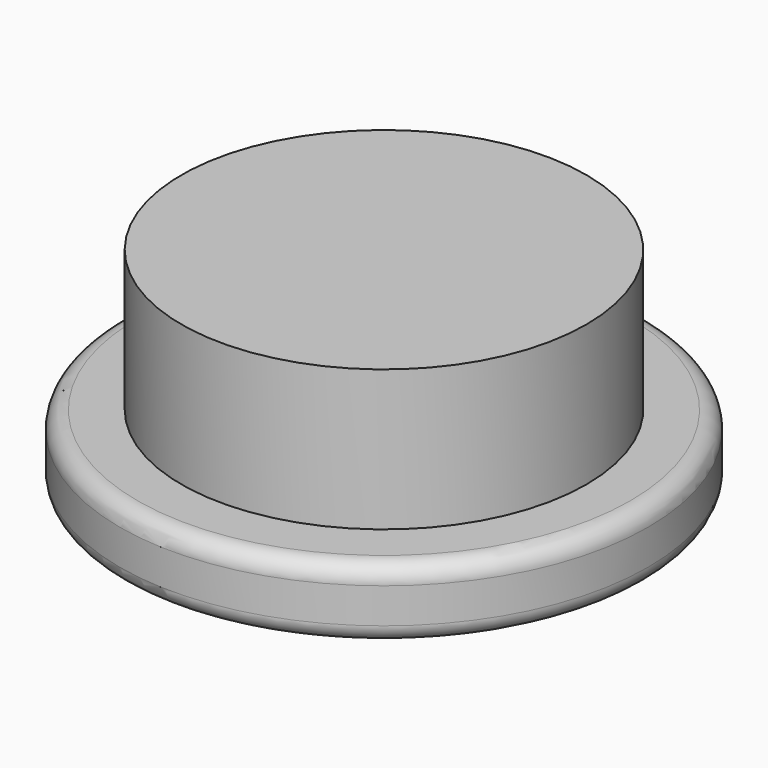
from build123d import *

# Parameters (mm, degrees)
F0_R     = 58.42
F1_DEPTH = 40.64
F2_R     = 76.2
F2_R_2   = 58.42
F3_DEPTH = 20.32
F4_R     = 5.08
F5_DEPTH = 17.78
F7_R     = 25.4
F8_DEPTH = 45.974


with BuildPart() as f1:
    # F0 (on Top) → F1 (new body)
    with BuildSketch(Plane.XY):
        with Locations((-23.1254743153, 3.4657202779)):
            Circle(F0_R)
    extrude(amount=F1_DEPTH)


with BuildPart() as f3:
    # F2 (on face) → F3 (new body)
    with BuildSketch(Plane(origin=(0, 0, 0), x_dir=(1, 0, 0), z_dir=(0, 0, -1))):
        with Locations((-23.1254743153, -3.4657202779)):
            Circle(F2_R)
        with Locations((-23.1254743153, -3.4657202779)):
            Circle(F2_R_2, mode=Mode.SUBTRACT)
    extrude(amount=F3_DEPTH)

    # F4
    f4_edges = [f3.edges().sort_by_distance(p)[0] for p in [
        (53.074526, 3.46572, -10.16),
        (-99.325474, 3.46572, 0),
        (-99.325474, 3.46572, -20.32),
    ]]
    fillet(f4_edges, radius=F4_R)


with BuildPart() as f5:
    # F5 (new): a face of the model
    f5_faces = [f1.part.faces().sort_by_distance(p)[0] for p in [
        (-23.1254743153, 3.4657202779, 0),
    ]]
    extrude(f5_faces, amount=F5_DEPTH)

    # F7 (on face) → F8 (cut)
    with BuildSketch(Plane(origin=(0, 0, -17.78), x_dir=(1, 0, 0), z_dir=(0, 0, -1))):
        with Locations((-22.6742904633, 0)):
            Circle(F7_R)
    extrude(amount=-F8_DEPTH, mode=Mode.SUBTRACT)


solid = Compound([f1.part, f3.part, f5.part])
